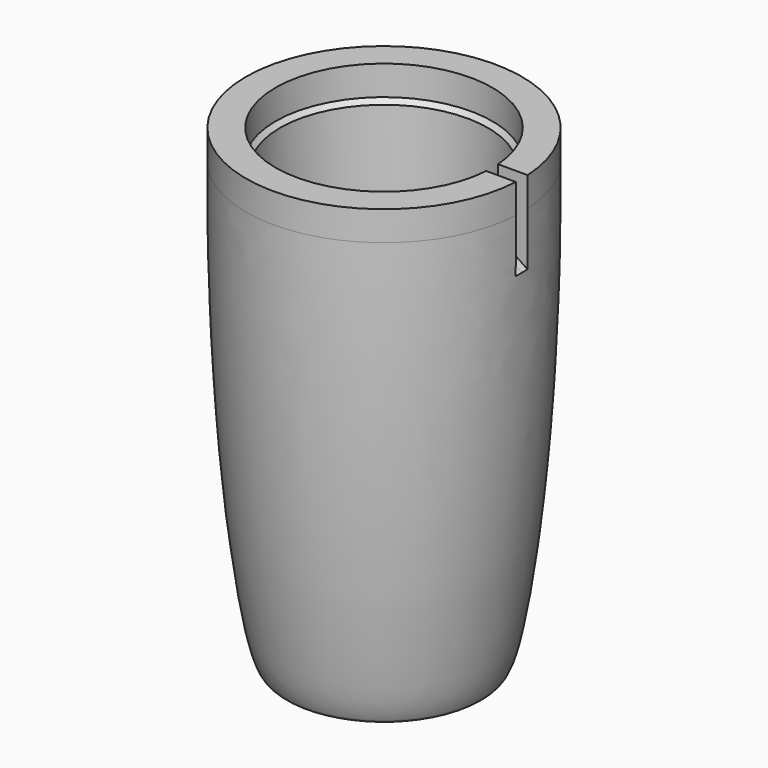
from build123d import *

# Parameters (mm, degrees)
F3_DEPTH    = 20
F4_T4_ANGLE = 41.1903305593
F4_T9_ANGLE = 41.1903607256


# Not quite as in the source:
# - a fillet or chamfer that OpenCascade refuses, or shapes differently, is made with other operations: its cross-section is extruded or revolved along the edge and cut away or added


with BuildPart() as f1:
    # F0 (on Front) → F1 (revolve)
    with BuildSketch(Plane.XZ):
        with BuildLine():
            Line((46.7, 0), (36.7, 0))
            Line((36.7, 0), (36.7, -10))
            Line((36.7, -10), (35.2, -11.5))
            Line((35.2, -11.5), (31.5, -160))
            add(Edge.make_bspline(
                [(31.5, -160), (34.9205158198, -163.1733860852), (45.1526020923, -104.4093913174), (46.8983203173, -37.4636948109), (46.7, -10)],
                knots=[0, 0, 0, 0, 0.3982770084, 1, 1, 1, 1], degree=3))
            Line((46.7, -10), (46.7, 0))
        make_face()
    revolve(axis=Axis((0, 0, -79.1394754779), (0, 0, -1)))

    # F2 (on face) → F3 (cut)
    with BuildSketch(Plane.XY):
        with BuildLine():
            ThreePointArc((46.6330355006, 2.5), (46.6832558734, 1.250448344), (46.7, 0))
            ThreePointArc((46.7, 0), (46.6832558734, -1.250448344), (46.6330355006, -2.5))
            Line((46.6330355006, -2.5), (51.9782938063, -2.5))
            Line((51.9782938063, -2.5), (51.9782938063, 2.5))
            Line((51.9782938063, 2.5), (46.6330355006, 2.5))
        make_face()
        with BuildLine():
            ThreePointArc((46.6330355006, -2.5), (46.6832558734, -1.250448344), (46.7, 0))
            ThreePointArc((46.7, 0), (46.6832558734, 1.250448344), (46.6330355006, 2.5))
            Line((46.6330355006, 2.5), (36.6147511257, 2.5))
            ThreePointArc((36.6147511257, 2.5), (36.6786815897, 1.2507265259), (36.7, 0))
            ThreePointArc((36.7, 0), (36.6786815897, -1.2507265259), (36.6147511257, -2.5))
            Line((36.6147511257, -2.5), (46.6330355006, -2.5))
        make_face()
        with BuildLine():
            ThreePointArc((36.7, 0), (36.6786815897, 1.2507265259), (36.6147511257, 2.5))
            Line((36.6147511257, 2.5), (32.3731712997, 2.5))
            Line((32.3731712997, 2.5), (32.3731712997, -2.5))
            Line((32.3731712997, -2.5), (36.6147511257, -2.5))
            ThreePointArc((36.6147511257, -2.5), (36.6786815897, -1.2507265259), (36.7, 0))
        make_face()
    extrude(amount=-F3_DEPTH, mode=Mode.SUBTRACT)

    # F4: chamfer of 12 x 8 on 2 edges, made by hand


with BuildPart() as f4_tool2:
    # F4_s3 → F4_t4 (revolve)
    with BuildSketch(Plane(origin=(-7.0888e-06, -8.1003e-06, 0), x_dir=(0, 0, 1), z_dir=(-0.6585624812, -0.7525260516, 0))):
        with BuildLine():
            Line((-28.3661524227, -47.0496779531), (-19.7310392649, -34.2855747254))
            Line((-19.7310392649, -34.2855747254), (-19.4910392649, -34.2855747254))
            ThreePointArc((-19.4910392649, -34.2855747254), (-19.76, -40.500764232), (-19.76, -46.7159537386))
            Line((-19.76, -46.7159537386), (-20.0009080776, -46.9559520207))
            ThreePointArc((-20.0009080776, -46.9559520207), (-24.1834649208, -46.9311818232), (-28.3690103838, -47.2896609359))
            Line((-28.3690103838, -47.2896609359), (-28.3661524227, -47.0496779531))
        make_face()
    revolve(axis=Axis((-1.71008e-05, 6.615e-07, -20), (0, 0, 1)), revolution_arc=F4_T4_ANGLE)

    split(bisect_by=Plane.XZ.offset(2.5), keep=Keep.BOTTOM)


with BuildPart() as f1_1:
    add(f1.part)

    # F4_t1: cut F4_tool2
    add(f4_tool2.part, mode=Mode.SUBTRACT)


with BuildPart() as f4_tool7:
    # F4_s8 → F4_t9 (revolve)
    with BuildSketch(Plane.XZ.offset(-2.542e-07)):
        with BuildLine():
            Line((47.0496741445, -28.3661524227), (34.2855709168, -19.7310392649))
            Line((34.2855709168, -19.7310392649), (34.2855709168, -19.4910392649))
            ThreePointArc((34.2855709168, -19.4910392649), (40.5007604241, -19.76), (46.7159499314, -19.76))
            Line((46.7159499314, -19.76), (46.9559482135, -20.0009080776))
            ThreePointArc((46.9559482135, -20.0009080776), (46.9311780146, -24.1834649208), (47.2896571273, -28.3690103838))
            Line((47.2896571273, -28.3690103838), (47.0496741445, -28.3661524227))
        make_face()
    revolve(axis=Axis((1.70968e-05, 2.542e-07, -20), (0, 0, 1)), revolution_arc=F4_T9_ANGLE)

    split(bisect_by=Plane.XZ.offset(-2.5), keep=Keep.TOP)


with BuildPart() as f1_2:
    add(f1_1.part)

    # F4_t6: cut F4_tool7
    add(f4_tool7.part, mode=Mode.SUBTRACT)


solid = f1_2.part
